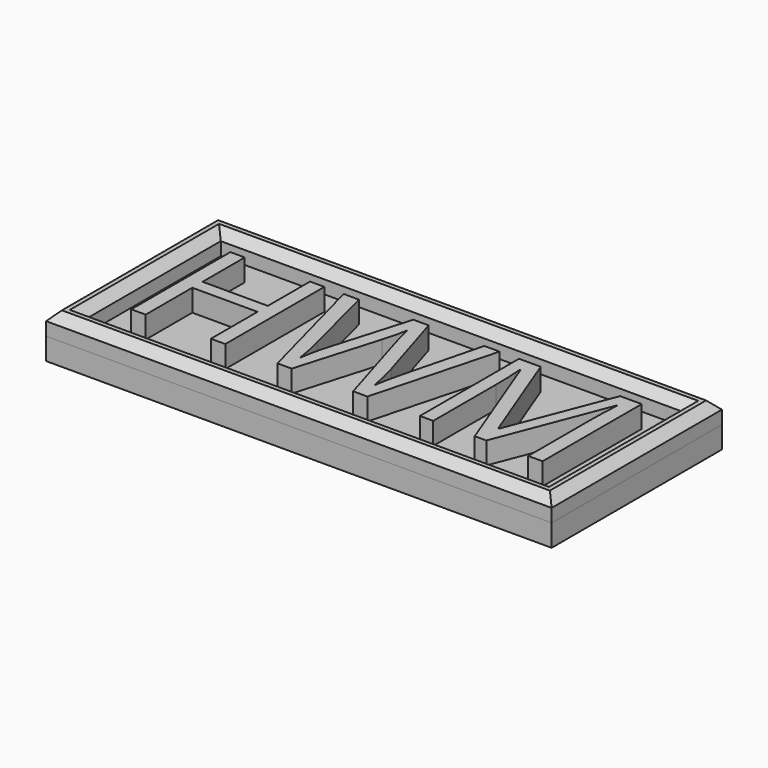
from build123d import *

# Parameters (mm, degrees)
F0_W         = 115
F0_H         = 48.418
F0_W_2       = 105
F0_H_2       = 38.418
F0_TEXT_SIZE = 39.4696268887
F1_DEPTH     = 5
F2_DEPTH     = 5
F3_SIZE      = 2
F4_W         = 21
F4_H         = 38.418
F5_DEPTH     = 0.75


# Not quite as in the source:
# - Text() gives the source's letters only with a copy of the font that has no kerning and outlines rounded to 1/6400 em; it was checked with that copy


with BuildPart() as f1:
    # F0 (on Top) → F1 (new body)
    with BuildSketch(Plane.XY):
        with Locations((-52.8948155046, -24.9578517888)):
            Rectangle(F0_W, F0_H)
        with Locations((-52.8948155046, -24.9578517888)):
            Rectangle(F0_W_2, F0_H_2, mode=Mode.SUBTRACT)
        with Locations((-102.8948155046, -39.1669174687)):
            Text('HWM', F0_TEXT_SIZE, font='Open Sans', text_align=(TextAlign.LEFT, TextAlign.BOTTOM))
    extrude(amount=F1_DEPTH)

    # F3
    f3_edges = [f1.edges().sort_by_distance(p)[0] for p in [
        (-110.394816, -24.957852, 5),
        (-52.894816, -0.748852, 5),
        (-52.894816, -5.748852, 5),
        (-105.394816, -24.957852, 5),
        (-52.894816, -44.166852, 5),
        (-52.894816, -49.166852, 5),
        (-0.394816, -24.957852, 5),
        (4.605184, -24.957852, 5),
    ]]
    chamfer(f3_edges, length=F3_SIZE)


with BuildPart() as f2:
    # F0 (on Top) → F2 (new body)
    with BuildSketch(Plane.XY):
        with Locations((-52.8948155046, -24.9578517888)):
            Rectangle(F0_W, F0_H)
        with Locations((-52.8948155046, -24.9578517888)):
            Rectangle(F0_W_2, F0_H_2, mode=Mode.SUBTRACT)
        with Locations((-52.8948155046, -24.9578517888)):
            Rectangle(F0_W_2, F0_H_2)
        Polygon((-77.6280871666, -10.9893041477), (-77.6280871666, -39.1669174687), (-80.9028327725, -39.1669174687), (-80.9028327725, -25.9075896858), (-95.7471127602, -25.9075896858), (-95.7471127602, -39.1669174687), (-99.0218583661, -39.1669174687), (-99.0218583661, -10.9893041477), (-95.7471127602, -10.9893041477), (-95.7471127602, -22.9782033151), (-80.9028327725, -22.9782033151), (-80.9028327725, -10.9893041477), align=None, mode=Mode.SUBTRACT)
        with BuildLine():
            Line((-37.7699311382, -10.9893041477), (-45.3061630223, -39.1669174687))
            Line((-45.3061630223, -39.1669174687), (-48.543905853, -39.1669174687))
            Line((-48.543905853, -39.1669174687), (-54.2299989766, -20.3016692417))
            add(Edge.make_bspline(
                [(-54.2299989766, -20.3016692417), (-54.6370295039, -19.0435748847), (-55.1365669692, -17.1379319614)],
                knots=[0, 0, 0, 1, 1, 1], degree=2))
            add(Edge.make_bspline(
                [(-55.1365669692, -17.1379319614), (-55.6361044346, -15.2322890382), (-55.6546058222, -14.8437598985)],
                knots=[0, 0, 0, 1, 1, 1], degree=2))
            add(Edge.make_bspline(
                [(-55.6546058222, -14.8437598985), (-56.0801377371, -17.3907842587), (-57.0052071173, -20.4126775674)],
                knots=[0, 0, 0, 1, 1, 1], degree=2))
            Line((-57.0052071173, -20.4126775674), (-62.5186206233, -39.1669174687))
            Line((-62.5186206233, -39.1669174687), (-65.756363454, -39.1669174687))
            Line((-65.756363454, -39.1669174687), (-73.2555925628, -10.9893041477))
            Line((-73.2555925628, -10.9893041477), (-69.7834988225, -10.9893041477))
            Line((-69.7834988225, -10.9893041477), (-65.3308315391, -28.3929427539))
            add(Edge.make_bspline(
                [(-65.3308315391, -28.3929427539), (-64.4057621589, -32.0562174995), (-63.980230244, -35.0226066454)],
                knots=[0, 0, 0, 1, 1, 1], degree=2))
            add(Edge.make_bspline(
                [(-63.980230244, -35.0226066454), (-63.4621913911, -31.4950087422), (-62.4384479437, -28.1215890691)],
                knots=[0, 0, 0, 1, 1, 1], degree=2))
            Line((-62.4384479437, -28.1215890691), (-57.3937362569, -10.9893041477))
            Line((-57.3937362569, -10.9893041477), (-53.9216425166, -10.9893041477))
            Line((-53.9216425166, -10.9893041477), (-48.6240785326, -28.2757672991))
            add(Edge.make_bspline(
                [(-48.6240785326, -28.2757672991), (-47.6990091524, -31.2668249617), (-47.0637948447, -35.0226066454)],
                knots=[0, 0, 0, 1, 1, 1], degree=2))
            add(Edge.make_bspline(
                [(-47.0637948447, -35.0226066454), (-46.6937670926, -32.28440128), (-45.6761907744, -28.3559399787)],
                knots=[0, 0, 0, 1, 1, 1], degree=2))
            Line((-45.6761907744, -28.3559399787), (-41.2420248786, -10.9893041477))
            Line((-41.2420248786, -10.9893041477), (-37.7699311382, -10.9893041477))
        make_face(mode=Mode.SUBTRACT)
        with BuildLine():
            Line((-18.2509672159, -39.1669174687), (-20.8904985141, -39.1669174687))
            Line((-20.8904985141, -39.1669174687), (-30.4495487762, -14.1900442032))
            Line((-30.4495487762, -14.1900442032), (-30.6037270062, -14.1900442032))
            add(Edge.make_bspline(
                [(-30.6037270062, -14.1900442032), (-30.3323733214, -17.156433349), (-30.3323733214, -21.2452400095)],
                knots=[0, 0, 0, 1, 1, 1], degree=2))
            Line((-30.3323733214, -21.2452400095), (-30.3323733214, -39.1669174687))
            Line((-30.3323733214, -39.1669174687), (-33.3604337593, -39.1669174687))
            Line((-33.3604337593, -39.1669174687), (-33.3604337593, -10.9893041477))
            Line((-33.3604337593, -10.9893041477), (-28.4267303982, -10.9893041477))
            Line((-28.4267303982, -10.9893041477), (-19.5028944438, -34.2332141076))
            Line((-19.5028944438, -34.2332141076), (-19.3487162138, -34.2332141076))
            Line((-19.3487162138, -34.2332141076), (-10.350874709, -10.9893041477))
            Line((-10.350874709, -10.9893041477), (-5.4541741231, -10.9893041477))
            Line((-5.4541741231, -10.9893041477), (-5.4541741231, -39.1669174687))
            Line((-5.4541741231, -39.1669174687), (-8.728919729, -39.1669174687))
            Line((-8.728919729, -39.1669174687), (-8.728919729, -21.0108890999))
            add(Edge.make_bspline(
                [(-8.728919729, -21.0108890999), (-8.728919729, -17.890321724), (-8.4575660442, -14.2270469784)],
                knots=[0, 0, 0, 1, 1, 1], degree=2))
            Line((-8.4575660442, -14.2270469784), (-8.6117442742, -14.2270469784))
            Line((-8.6117442742, -14.2270469784), (-18.2509672159, -39.1669174687))
        make_face(mode=Mode.SUBTRACT)
        with Locations((-102.8948155046, -39.1669174687)):
            Text('HWM', F0_TEXT_SIZE, font='Open Sans', text_align=(TextAlign.LEFT, TextAlign.BOTTOM))
    extrude(amount=-F2_DEPTH)

    # F4 (on face) → F5 (cut)
    with BuildSketch(Plane(origin=(0, 0, -5), x_dir=(1, 0, 0), z_dir=(0, 0, -1))):
        with Locations((-94.8948155046, 24.9578517888)):
            Rectangle(F4_W, F4_H)
        with Locations((-10.8948155046, 24.9578517888)):
            Rectangle(F4_W, F4_H)
    extrude(amount=-F5_DEPTH, mode=Mode.SUBTRACT)


solid = Compound([f1.part, f2.part])
